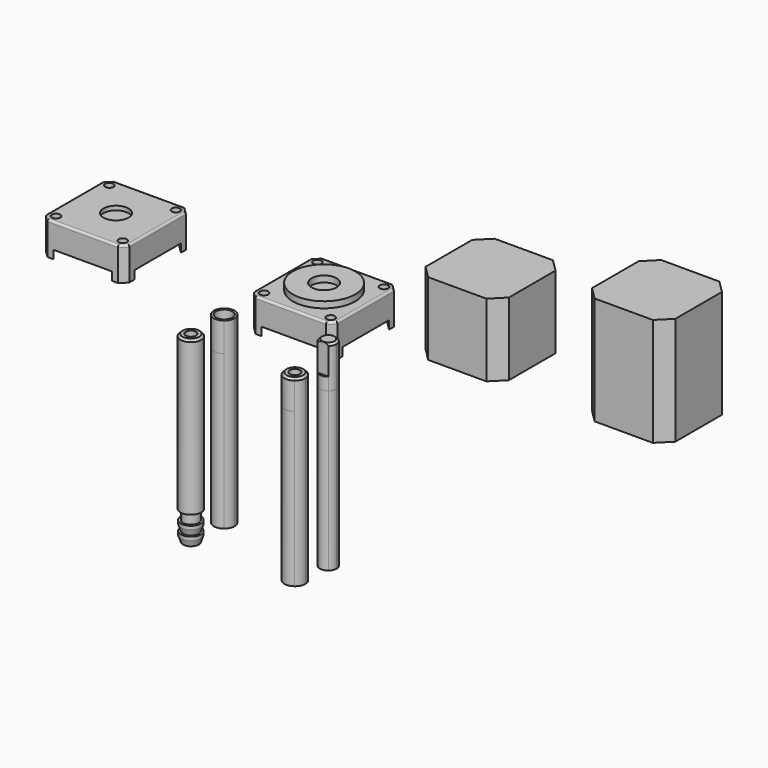
from build123d import *

# Parameters (mm, degrees)
F0_R         = 3
F1_DEPTH     = 6
F0_R_2       = 7.5
F2_DEPTH     = 1.5
F3_DEPTH     = 1
F5_DEPTH     = 2
F6_D         = 2
F6_DEPTH     = 3
F6_TIP       = 0.600860619
F6_2_D       = 2
F6_2_DEPTH   = 3
F6_2_TIP     = 0.600860619
F7_DEPTH     = 17.5
F8_DEPTH     = 7
F9_R         = 0.5
F9_2_R       = 0.5
F10_SIZE     = 0.5
F10_2_SIZE   = 0.5
F11_DEPTH    = 37
F12_R        = 1.25
F12_R_2      = 2
F13_DEPTH    = 44.001
F16_DEPTH    = 26
F18_DEPTH    = 10
F20_DEPTH    = 7
F21_T2_ANGLE = 317.2277824927
F21_T4_ANGLE = 137.0086765411
F22_DEPTH    = 38


# Not quite as in the source:
# - a fillet or chamfer that OpenCascade refuses, or shapes differently, is made with other operations: its cross-section is extruded or revolved along the edge and cut away or added


with BuildPart() as f1:
    # F0 (on Top) → F1 (new body)
    with BuildSketch(Plane.XY):
        Polygon((-60, 7), (-60, -7), (-57, -10), (-43, -10), (-40, -7), (-40, 7), (-43, 10), (-57, 10), align=None)
        with Locations((-50, 0)):
            Circle(F0_R, mode=Mode.SUBTRACT)
        Polygon((-41.5, 10), (-43, 10), (-40, 7), (-40, 8.5), align=None)
        Polygon((-60, 8.5), (-60, 7), (-57, 10), (-58.5, 10), align=None)
        Polygon((-60, -7), (-60, -8.5), (-58.5, -10), (-57, -10), align=None)
        Polygon((-40, -7), (-43, -10), (-41.5, -10), (-40, -8.5), align=None)
        with Locations((-50, 0)):
            Circle(F0_R)
    extrude(amount=-F1_DEPTH)

    # F0 (on Top) → F3 (cut)
    with BuildSketch(Plane.XY):
        with Locations((-50, 0)):
            Circle(F0_R)
    extrude(amount=-F3_DEPTH, mode=Mode.SUBTRACT)

    # F4 (on face) → F5 (join)
    with BuildSketch(Plane(origin=(0, 0, -6), x_dir=(1, 0, 0), z_dir=(0, 0, -1))):
        Polygon((-40, -7), (-43, -10), (-41.5, -10), (-40, -8.5), align=None)
        Polygon((-58.5, -10), (-57, -10), (-60, -7), (-60, -8.5), align=None)
        Polygon((-60, 7), (-57, 10), (-58.5, 10), (-60, 8.5), align=None)
        Polygon((-40, 7), (-40, 8.5), (-41.5, 10), (-43, 10), align=None)
    extrude(amount=F5_DEPTH)

    # F6
    with Locations(Plane.XY):
        with Locations((-8, -8), (8, -8), (8, 8), (-8, 8), (-42, -8), (-42, 8), (-58, 8), (-58, -8)):
            Hole(F6_D / 2, depth=F6_DEPTH)
            with Locations((0, 0, -(F6_DEPTH + F6_TIP / 2))):  # 118° drill point
                Cone(0, F6_D / 2, F6_TIP, mode=Mode.SUBTRACT)

    # F9
    f9_edges = [f1.edges().sort_by_distance(p)[0] for p in [
        (-40, 0, 0),
        (-40.75, -9.25, 0),
        (-59.25, -9.25, 0),
        (-60, 0, 0),
        (-50, -10, 0),
        (-50, 10, 0),
        (-40.75, 9.25, 0),
        (-59.25, 9.25, 0),
    ]]
    fillet(f9_edges, radius=F9_R)


with BuildPart() as f1b:
    # F0 (on Top) → F1, piece 2 (new body)
    with BuildSketch(Plane.XY):
        Polygon((-7, -10), (7, -10), (10, -7), (10, 7), (7, 10), (-7, 10), (-10, 7), (-10, -7), align=None)
        Circle(F0_R_2, mode=Mode.SUBTRACT)
        Circle(F0_R_2)
        Circle(F0_R, mode=Mode.SUBTRACT)
        Polygon((-8.5, -10), (-7, -10), (-10, -7), (-10, -8.5), align=None)
        Polygon((-10, 8.5), (-10, 7), (-7, 10), (-8.5, 10), align=None)
        Polygon((7, 10), (10, 7), (10, 8.5), (8.5, 10), align=None)
        Polygon((7, -10), (8.5, -10), (10, -8.5), (10, -7), align=None)
        Circle(F0_R)
    extrude(amount=-F1_DEPTH)

    # F0 (on Top) → F2 (join)
    with BuildSketch(Plane.XY):
        Circle(F0_R_2)
        Circle(F0_R, mode=Mode.SUBTRACT)
    extrude(amount=F2_DEPTH)

    # F4 (on face) → F5, piece 2 (join)
    with BuildSketch(Plane(origin=(0, 0, -6), x_dir=(1, 0, 0), z_dir=(0, 0, -1))):
        Polygon((-8.5, -10), (-7, -10), (-10, -7), (-10, -8.5), align=None)
        Polygon((10, -7), (7, -10), (8.5, -10), (10, -8.5), align=None)
        Polygon((7, 10), (10, 7), (10, 8.5), (8.5, 10), align=None)
        Polygon((-10, 8.5), (-10, 7), (-7, 10), (-8.5, 10), align=None)
    extrude(amount=F5_DEPTH)

    # F6#2
    with Locations(Plane.XY):
        with Locations((-8, -8), (8, -8), (8, 8), (-8, 8), (-42, -8), (-42, 8), (-58, 8), (-58, -8)):
            Hole(F6_2_D / 2, depth=F6_2_DEPTH)
            with Locations((0, 0, -(F6_2_DEPTH + F6_2_TIP / 2))):  # 118° drill point
                Cone(0, F6_2_D / 2, F6_2_TIP, mode=Mode.SUBTRACT)

    # F9#2
    f9_2_edges = [f1b.edges().sort_by_distance(p)[0] for p in [
        (-10, 0, 0),
        (-9.25, -9.25, 0),
        (0, -10, 0),
        (9.25, -9.25, 0),
        (10, 0, 0),
        (9.25, 9.25, 0),
        (0, 10, 0),
        (-9.25, 9.25, 0),
    ]]
    fillet(f9_2_edges, radius=F9_2_R)


with BuildPart() as f7:
    # F0 (on Top) → F7 (new body)
    with BuildSketch(Plane.XY):
        Polygon((33, -10), (47, -10), (50, -7), (50, 7), (47, 10), (33, 10), (30, 7), (30, -7), align=None)
    extrude(amount=F7_DEPTH)


with BuildPart() as f8:
    # F0 (on Top) → F8 (new body)
    with BuildSketch(Plane.XY):
        with BuildLine():
            ThreePointArc((1.5, -32), (2.2360679775, -31.1180339887), (2.5, -30))
            ThreePointArc((2.5, -30), (-1.1180339887, -27.7639320225), (-1.5, -32))
            Line((-1.5, -32), (1.5, -32))
        make_face()
        with BuildLine():
            Line((1.5, -32), (-1.5, -32))
            ThreePointArc((-1.5, -32), (0, -32.5), (1.5, -32))
        make_face()
    extrude(amount=F8_DEPTH)

    # F11#2 (add): a face of the model
    f11_2_faces = [f8.faces().sort_by_distance(p)[0] for p in [
        (0, -30, 0),
    ]]
    extrude(f11_2_faces, amount=F11_DEPTH)


with BuildPart() as f8b:
    # F0 (on Top) → F8, piece 2 (new body)
    with BuildSketch(Plane.XY):
        with BuildLine():
            ThreePointArc((1.5, -42), (2.2360679775, -41.1180339887), (2.5, -40))
            ThreePointArc((2.5, -40), (-1.1180339887, -37.7639320225), (-1.5, -42))
            Line((-1.5, -42), (1.5, -42))
        make_face()
        with BuildLine():
            Line((1.5, -42), (-1.5, -42))
            ThreePointArc((-1.5, -42), (0, -42.5), (1.5, -42))
        make_face()
    extrude(amount=F8_DEPTH)

    # F10
    f10_edges = [f8b.edges().sort_by_distance(p)[0] for p in [
        (-2.5, -40, 7),
    ]]
    chamfer(f10_edges, length=F10_SIZE)

    # F11 (add): a face of the model
    f11_faces = [f8b.faces().sort_by_distance(p)[0] for p in [
        (0, -40, 0),
    ]]
    extrude(f11_faces, amount=F11_DEPTH)


with BuildPart() as f8c:
    # F0 (on Top) → F8, piece 3 (new body)
    with BuildSketch(Plane.XY):
        with BuildLine():
            ThreePointArc((26.5, -42), (27.2360679775, -41.1180339887), (27.5, -40))
            ThreePointArc((27.5, -40), (23.8819660113, -37.7639320225), (23.5, -42))
            Line((23.5, -42), (26.5, -42))
        make_face()
        with BuildLine():
            Line((26.5, -42), (23.5, -42))
            ThreePointArc((23.5, -42), (25, -42.5), (26.5, -42))
        make_face()
    extrude(amount=F8_DEPTH)

    # F10#2
    f10_2_edges = [f8c.edges().sort_by_distance(p)[0] for p in [
        (22.5, -40, 7),
    ]]
    chamfer(f10_2_edges, length=F10_2_SIZE)

    # F11#3 (add): a face of the model
    f11_3_faces = [f8c.faces().sort_by_distance(p)[0] for p in [
        (25, -40, 0),
    ]]
    extrude(f11_3_faces, amount=F11_DEPTH)


with BuildPart() as f13_tool:
    # F12 (on face) → F13 (new body, through all)
    with BuildSketch(Plane.XY.offset(7)):
        with Locations((0, -40)):
            Circle(F12_R)
        with Locations((0, -30)):
            Circle(F12_R_2)
        with Locations((25, -40)):
            Circle(F12_R)
    extrude(amount=-F13_DEPTH)


with BuildPart() as f8_1:
    add(f8.part)

    # F13: cut by f13_tool
    add(f13_tool.part, mode=Mode.SUBTRACT)


with BuildPart() as f8b_1:
    add(f8b.part)

    # F13: cut by f13_tool
    add(f13_tool.part, mode=Mode.SUBTRACT)

    # F14 (on Right) → F15 (revolve, cut)
    with BuildSketch(Plane.YZ):
        Polygon((-42.5, -30), (-42.5, -32.4), (-42.4, -32.4), (-41.9, -32.4), (-41.9, -30), align=None)
        Polygon((-42.5, -32.4), (-42.5, -37), (-41.9, -37), (-42.4, -35.5), (-42.4, -34.7), (-41.9, -34.7), (-42.4, -33.2), (-42.4, -32.4), align=None)
    revolve(axis=Axis((0, -40, -33.5), (0, 0, 1)), mode=Mode.SUBTRACT)


with BuildPart() as f8c_1:
    add(f8c.part)

    # F13: cut by f13_tool
    add(f13_tool.part, mode=Mode.SUBTRACT)


with BuildPart() as f16:
    # F0 (on Top) → F16 (new body)
    with BuildSketch(Plane.XY):
        Polygon((73, -10), (87, -10), (90, -7), (90, 7), (87, 10), (73, 10), (70, 7), (70, -7), align=None)
    extrude(amount=F16_DEPTH)


with BuildPart() as f18:
    # F17 (on Top) → F18 (new body)
    with BuildSketch(Plane.XY):
        with BuildLine():
            ThreePointArc((26.3228756555, -31.5), (26.8228756555, -30.8228756555), (27, -30))
            ThreePointArc((27, -30), (24.1771243445, -28.1771243445), (23.6771243445, -31.5))
            Line((23.6771243445, -31.5), (26.3228756555, -31.5))
        make_face()
        with BuildLine():
            Line((26.3228756555, -31.5), (23.6771243445, -31.5))
            ThreePointArc((23.6771243445, -31.5), (25, -32), (26.3228756555, -31.5))
        make_face()
    extrude(amount=F18_DEPTH)

    # F19 (on face) → F20 (cut)
    with BuildSketch(Plane.XY.offset(10)):
        with BuildLine():
            Line((26.3228756555, -31.5), (23.6771243445, -31.5))
            ThreePointArc((23.6771243445, -31.5), (25, -32), (26.3228756555, -31.5))
        make_face()
    extrude(amount=-F20_DEPTH, mode=Mode.SUBTRACT)

    # F21: chamfer of 0.5 on 2 edges, made by hand

    # F21_s1 → F21_t2 (revolve, cut)
    with BuildSketch(Plane.XZ.offset(30)):
        with BuildLine():
            Line((27.0141421356, 9.4858578644), (26.4858578644, 10.0141421356))
            Line((26.4858578644, 10.0141421356), (26.4858578644, 10.0241421356))
            ThreePointArc((26.4858578644, 10.0241421356), (26.7429289322, 10.01), (27, 10.01))
            Line((27, 10.01), (27.01, 10))
            ThreePointArc((27.01, 10), (27.01, 9.7429289322), (27.0241421356, 9.4858578644))
            Line((27.0241421356, 9.4858578644), (27.0141421356, 9.4858578644))
        make_face()
    revolve(axis=Axis((25, -30, 10), (0, 0, 1)), revolution_arc=F21_T2_ANGLE, mode=Mode.SUBTRACT)

    # F21_s3 → F21_t4 (revolve, cut)
    with BuildSketch(Plane(origin=(26.5874106472, -28.5201649863, 0), x_dir=(0, 0, 1), z_dir=(-0.6818876003, 0.7314569711, 0))):
        with BuildLine():
            Line((9.4858578644, -4.1843458659), (10.0141421356, -3.6560615946))
            Line((10.0141421356, -3.6560615946), (10.0241421356, -3.6560615946))
            ThreePointArc((10.0241421356, -3.6560615946), (10.01, -3.9131326625), (10.01, -4.1702037303))
            Line((10.01, -4.1702037303), (10, -4.1802037303))
            ThreePointArc((10, -4.1802037303), (9.7429289322, -4.1802037303), (9.4858578644, -4.1943458659))
            Line((9.4858578644, -4.1943458659), (9.4858578644, -4.1843458659))
        make_face()
    revolve(axis=Axis((25, -30, 10), (0, 0, 1)), revolution_arc=F21_T4_ANGLE, mode=Mode.SUBTRACT)

    # F17 (on Top) → F22 (join)
    with BuildSketch(Plane.XY):
        with BuildLine():
            ThreePointArc((26.3228756555, -31.5), (26.8228756555, -30.8228756555), (27, -30))
            ThreePointArc((27, -30), (24.1771243445, -28.1771243445), (23.6771243445, -31.5))
            Line((23.6771243445, -31.5), (26.3228756555, -31.5))
        make_face()
        with BuildLine():
            Line((26.3228756555, -31.5), (23.6771243445, -31.5))
            ThreePointArc((23.6771243445, -31.5), (25, -32), (26.3228756555, -31.5))
        make_face()
    extrude(amount=-F22_DEPTH)


solid = Compound([f1.part, f1b.part, f7.part, f8_1.part, f8b_1.part, f8c_1.part, f16.part, f18.part])
